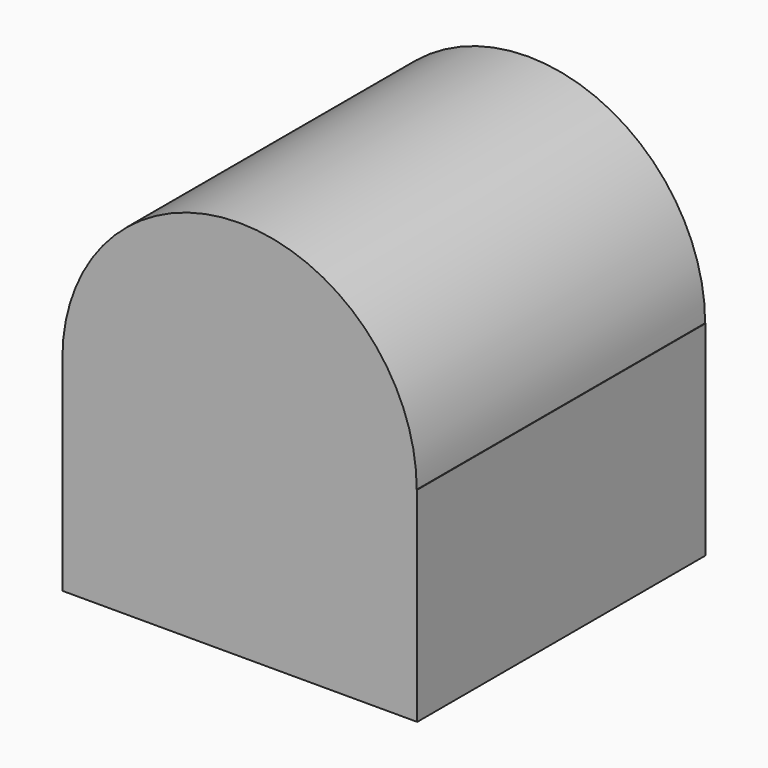
from build123d import *

# Parameters (mm, degrees)
F1_DEPTH = 97.6482406259


# Not quite as in the source:
# - the program builds the solid bodies; features that only make, move or delete a surface that nothing else refers to are left out


with BuildPart() as f1:
    # F0 (on Front) → F1 (new body)
    with BuildSketch(Plane.XZ):
        Polygon((47.9935407639, 0), (-47.9935407639, 0), (-47.9935407639, -55.3510189056), (48.1260120869, -55.3510189056), (48.1260120869, 0), align=None)
        with BuildLine():
            ThreePointArc((47.9935407639, 0), (0, 47.9935407639), (-47.9935407639, 0))
            Line((-47.9935407639, 0), (47.9935407639, 0))
        make_face()
    extrude(amount=F1_DEPTH)


solid = f1.part
